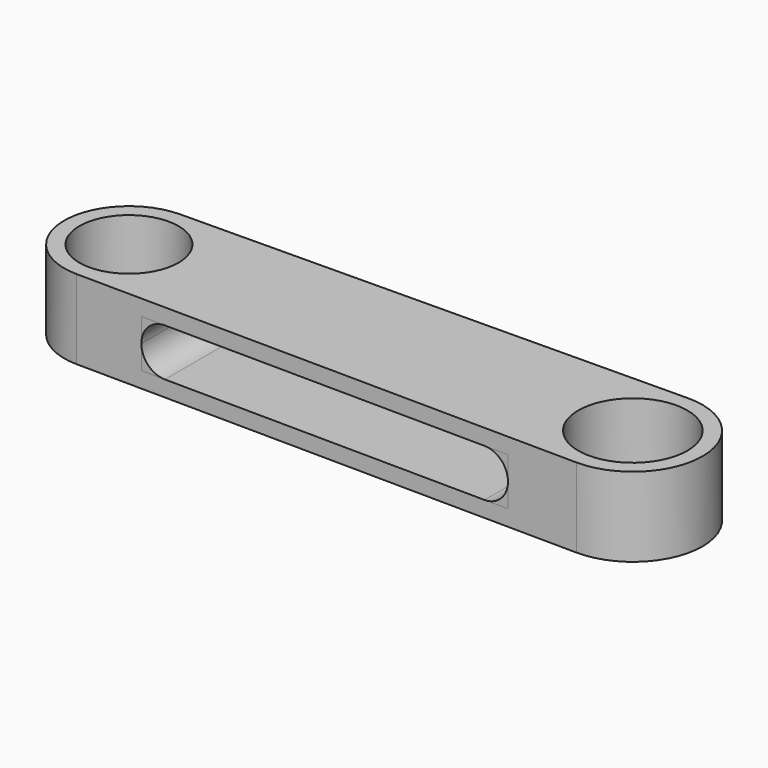
from build123d import *

# Parameters (mm, degrees)
F0_R          = 5.5
F0_R_2        = 5
F2_DEPTH      = 4
F3_W          = 37.252
F3_H          = 4.7996
F4_DEPTH      = 7.025
F4_DEPTH_BACK = 7.025
F5_T4_DEPTH   = 25.1150634776
F5_T10_DEPTH  = 25.1150634776
F5_T16_DEPTH  = 25.8484060864
F5_T22_DEPTH  = 25.8484060864


# Not quite as in the source:
# - a fillet or chamfer that OpenCascade refuses, or shapes differently, is made with other operations: its cross-section is extruded or revolved along the edge and cut away or added


with BuildPart() as f2:
    # F0 (on Top) → F2 (new body, symmetric)
    with BuildSketch(Plane.XY):
        with BuildLine():
            ThreePointArc((-25.4642125984, 6.5236839855), (-20.8095940807, 4.6358116329), (-18.876, 0))
            ThreePointArc((-18.876, 0), (-20.8095940807, -4.6358116329), (-25.4642125984, -6.5236839855))
            Line((-25.4642125984, -6.5236839855), (25.3308661417, -7.0236597661))
            ThreePointArc((25.3308661417, -7.0236597661), (18.376, 0), (25.3308661417, 7.0236597661))
            Line((25.3308661417, 7.0236597661), (-25.4642125984, 6.5236839855))
        make_face()
        with BuildLine():
            ThreePointArc((32.424, 0), (30.3422150793, 4.9911006913), (25.3308661417, 7.0236597661))
            ThreePointArc((25.3308661417, 7.0236597661), (18.376, 0), (25.3308661417, -7.0236597661))
            ThreePointArc((25.3308661417, -7.0236597661), (30.3422150793, -4.9911006913), (32.424, 0))
        make_face()
        with Locations((25.4, 0)):
            Circle(F0_R, mode=Mode.SUBTRACT)
        with BuildLine():
            ThreePointArc((-25.4642125984, -6.5236839855), (-20.8095940807, -4.6358116329), (-18.876, 0))
            ThreePointArc((-18.876, 0), (-20.8095940807, 4.6358116329), (-25.4642125984, 6.5236839855))
            ThreePointArc((-25.4642125984, 6.5236839855), (-31.924, 0), (-25.4642125984, -6.5236839855))
        make_face()
        with Locations((-25.4, 0)):
            Circle(F0_R_2, mode=Mode.SUBTRACT)
    extrude(amount=F2_DEPTH, both=True)

    # F3 (on Front) → F4 (cut, two sides)
    with BuildSketch(Plane.XZ) as f4_sk:
        with Locations((-0.25, 0)):
            Rectangle(F3_W, F3_H)
    extrude(amount=-F4_DEPTH, mode=Mode.SUBTRACT)
    extrude(f4_sk.sketch, amount=F4_DEPTH_BACK, mode=Mode.SUBTRACT)

    # F5: fillet of radius 2.3876 on 4 edges, made by hand


with BuildPart() as f5_tool2:
    # F5_s3 → F5_t4 (new body)
    with BuildSketch(Plane.XZ.offset(-12.5575317388)):
        with BuildLine():
            ThreePointArc((-18.876, 0.0122), (-18.1766881508, 1.7004881508), (-16.4884, 2.3998))
            Line((-16.4884, 2.3998), (-18.876, 2.3998))
            Line((-18.876, 2.3998), (-18.876, 0.0122))
        make_face()
    extrude(amount=F5_T4_DEPTH)

    split(bisect_by=Plane(origin=(-0.0666732283, 6.7736718758, 0), x_dir=(0, 0, 1), z_dir=(0.0098425197, -0.9999515612, 0)), keep=Keep.TOP)

    split(bisect_by=Plane(origin=(-0.0666732283, -6.7736718758, 0), x_dir=(0, 0, 1), z_dir=(0.0098425197, 0.9999515612, 0)), keep=Keep.TOP)


with BuildPart() as f2_1:
    add(f2.part)

    # F5_t1: union F5_tool2
    add(f5_tool2.part)


with BuildPart() as f5_tool8:
    # F5_s9 → F5_t10 (new body)
    with BuildSketch(Plane.XZ.offset(12.5575317388)):
        with BuildLine():
            ThreePointArc((-16.4884, -2.3998), (-18.1766881508, -1.7004881508), (-18.876, -0.0122))
            Line((-18.876, -0.0122), (-18.876, -2.3998))
            Line((-18.876, -2.3998), (-16.4884, -2.3998))
        make_face()
    extrude(amount=-F5_T10_DEPTH)

    split(bisect_by=Plane(origin=(-0.0666732283, 6.7736718758, 0), x_dir=(0, 0, 1), z_dir=(0.0098425197, -0.9999515612, 0)), keep=Keep.TOP)

    split(bisect_by=Plane(origin=(-0.0666732283, -6.7736718758, 0), x_dir=(0, 0, 1), z_dir=(0.0098425197, 0.9999515612, 0)), keep=Keep.TOP)


with BuildPart() as f2_2:
    add(f2_1.part)

    # F5_t7: union F5_tool8
    add(f5_tool8.part)


with BuildPart() as f5_tool14:
    # F5_s15 → F5_t16 (new body)
    with BuildSketch(Plane.XZ.offset(12.9242030432)):
        with BuildLine():
            ThreePointArc((18.376, -0.0122), (17.6766881508, -1.7004881508), (15.9884, -2.3998))
            Line((15.9884, -2.3998), (18.376, -2.3998))
            Line((18.376, -2.3998), (18.376, -0.0122))
        make_face()
    extrude(amount=-F5_T16_DEPTH)

    split(bisect_by=Plane(origin=(-0.0666732283, 6.7736718758, 0), x_dir=(0, 0, 1), z_dir=(0.0098425197, -0.9999515612, 0)), keep=Keep.TOP)

    split(bisect_by=Plane(origin=(-0.0666732283, -6.7736718758, 0), x_dir=(0, 0, 1), z_dir=(0.0098425197, 0.9999515612, 0)), keep=Keep.TOP)


with BuildPart() as f2_3:
    add(f2_2.part)

    # F5_t13: union F5_tool14
    add(f5_tool14.part)


with BuildPart() as f5_tool20:
    # F5_s21 → F5_t22 (new body)
    with BuildSketch(Plane.XZ.offset(-12.9242030432)):
        with BuildLine():
            ThreePointArc((18.376, 0.0122), (17.6766881508, 1.7004881508), (15.9884, 2.3998))
            Line((15.9884, 2.3998), (18.376, 2.3998))
            Line((18.376, 2.3998), (18.376, 0.0122))
        make_face()
    extrude(amount=F5_T22_DEPTH)

    split(bisect_by=Plane(origin=(-0.0666732283, 6.7736718758, 0), x_dir=(0, 0, 1), z_dir=(0.0098425197, -0.9999515612, 0)), keep=Keep.TOP)

    split(bisect_by=Plane(origin=(-0.0666732283, -6.7736718758, 0), x_dir=(0, 0, 1), z_dir=(0.0098425197, 0.9999515612, 0)), keep=Keep.TOP)


with BuildPart() as f2_4:
    add(f2_3.part)

    # F5_t19: union F5_tool20
    add(f5_tool20.part)


solid = f2_4.part
